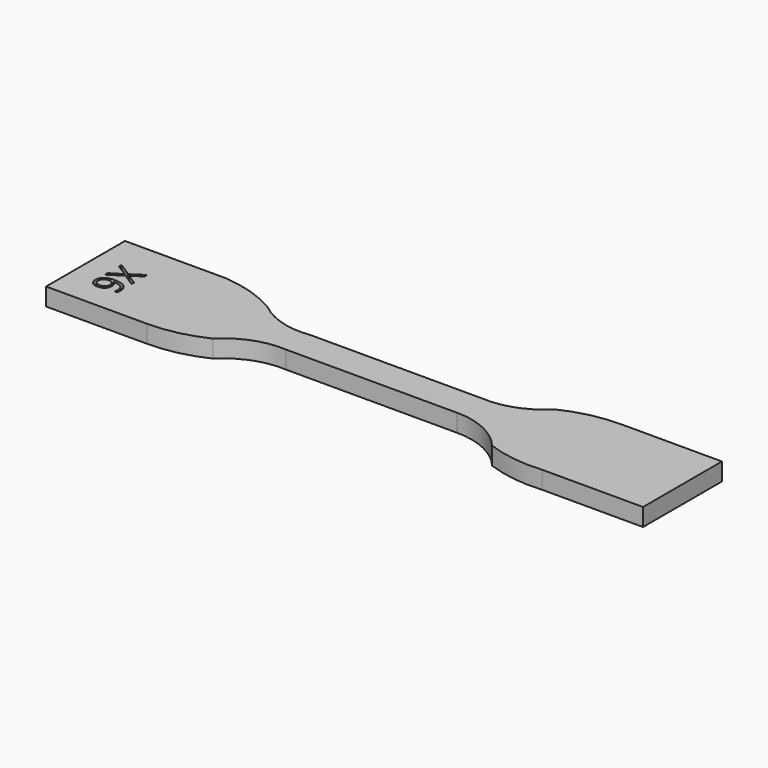
from build123d import *

# Parameters (mm, degrees)
F1_DEPTH     = 3.4
F2_TEXT_SIZE = 7.0564552314
F3_DEPTH     = 1


# Not quite as in the source:
# - Text() gives the source's letters only with a copy of the font that has no kerning and outlines rounded to 1/6400 em; it was checked with that copy


with BuildPart() as f1:
    # F0 (on Top) → F1 (new body)
    with BuildSketch(Plane.XY):
        with BuildLine():
            Line((-14.4320548165, 19.7811394548), (-33.8720548165, 19.7811394548))
            Line((-33.8720548165, 19.7811394548), (-33.8720548165, 0.7811394548))
            Line((-33.8720548165, 0.7811394548), (-14.4320548165, 0.7811394548))
            ThreePointArc((-14.4320548165, 0.7811394548), (-8.9053122052, 1.3996892086), (-3.6520548165, 3.2247301661))
            ThreePointArc((-3.6520548165, 3.2247301661), (1.3014698263, 6.4128780055), (7.1279451835, 7.2811394548))
            Line((7.1279451835, 7.2811394548), (40.1279451835, 7.2811394548))
            ThreePointArc((40.1279451835, 7.2811394548), (46.0837574042, 5.9511158081), (50.9079451835, 2.2137538538))
            ThreePointArc((50.9079451835, 2.2137538538), (56.2191047011, 0.9041953221), (61.6879451835, 0.7811394548))
            Line((61.6879451835, 0.7811394548), (81.1279451835, 0.7811394548))
            Line((81.1279451835, 0.7811394548), (81.1279451835, 19.7811394548))
            Line((81.1279451835, 19.7811394548), (61.6879451835, 19.7811394548))
            ThreePointArc((61.6879451835, 19.7811394548), (56.1612025723, 19.162589701), (50.9079451835, 17.3375487435))
            ThreePointArc((50.9079451835, 17.3375487435), (45.9544205407, 14.1494009041), (40.1279451835, 13.2811394548))
            Line((40.1279451835, 13.2811394548), (7.1279451835, 13.2811394548))
            ThreePointArc((7.1279451835, 13.2811394548), (1.4167452884, 13.6925537245), (-3.6520548165, 16.3560723447))
            ThreePointArc((-3.6520548165, 16.3560723447), (-8.8458057958, 18.686276846), (-14.4320548165, 19.7811394548))
        make_face()
    extrude(amount=F1_DEPTH)

    # F2 (on face) → F3 (cut)
    with BuildSketch(Plane.XY.offset(3.4)):
        with Locations(Location((-29.3720550835, 13.353464842), (0, 0, -90))):
            Text('X6', F2_TEXT_SIZE, font='Open Sans', text_align=(TextAlign.LEFT, TextAlign.BOTTOM))
    extrude(amount=-F3_DEPTH, mode=Mode.SUBTRACT)


solid = f1.part
